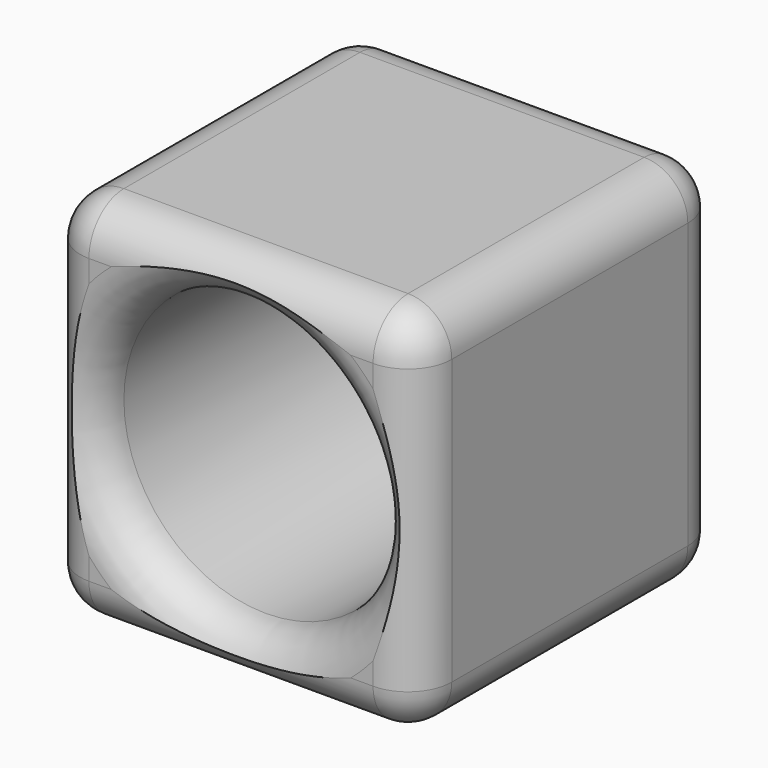
from build123d import *

# Parameters (mm, degrees)
F0_R         = 16.51
F1_DEPTH     = 6.35
F2_DEPTH     = 44.45
F3_T1_DEPTH  = 34.29
F3_T3_DEPTH  = 33.02
F3_T5_DEPTH  = 33.02
F3_S9_W      = 5.08
F3_S9_H      = 5.08
F3_T10_DEPTH = 5.08
F3_S15_W     = 5.08
F3_S15_H     = 5.08
F3_T16_DEPTH = 5.08
F3_S21_W     = 5.08
F3_S21_H     = 5.08
F3_T22_DEPTH = 5.08
F3_S27_W     = 5.08
F3_S27_H     = 5.08
F3_T28_DEPTH = 5.08
F3_S33_W     = 5.08
F3_S33_H     = 5.08
F3_T34_DEPTH = 5.08
F3_S39_W     = 5.08
F3_S39_H     = 5.08
F3_T40_DEPTH = 5.08
F3_S45_W     = 5.08
F3_S45_H     = 5.08
F3_T46_DEPTH = 5.08
F3_S51_W     = 5.08
F3_S51_H     = 5.08
F3_T52_DEPTH = 5.08
F4_R         = 3.175
F5_DEPTH     = 25.4


# Not quite as in the source:
# - a fillet or chamfer that OpenCascade refuses, or shapes differently, is made with other operations: its cross-section is extruded or revolved along the edge and cut away or added


with BuildPart() as f1:
    # F0 (on Front) → F1 (new body)
    with BuildSketch(Plane.XZ):
        Circle(F0_R)
    extrude(amount=F1_DEPTH)

    # F0 (on Front) → F2 (join)
    with BuildSketch(Plane.XZ):
        Polygon((21.59, 21.59), (0, 21.59), (-21.59, 21.59), (-21.59, 0), (-21.59, -21.59), (21.59, -21.59), align=None)
        Circle(F0_R, mode=Mode.SUBTRACT)
    extrude(amount=F2_DEPTH)

    # F3: fillet of radius 5.08 on 13 edges, made by hand

    # F3_s2 → F3_t1 (cut)
    with BuildSketch(Plane.XZ.offset(5.08)):
        with BuildLine():
            ThreePointArc((16.51, 21.59), (20.1021024484, 20.1021024484), (21.59, 16.51))
            Line((21.59, 16.51), (21.59, 21.59))
            Line((21.59, 21.59), (16.51, 21.59))
        make_face()
        with BuildLine():
            ThreePointArc((-16.51, 21.59), (-20.1021024484, 20.1021024484), (-21.59, 16.51))
            Line((-21.59, 16.51), (-21.59, 21.59))
            Line((-21.59, 21.59), (-16.51, 21.59))
        make_face()
        with BuildLine():
            ThreePointArc((-21.59, -16.51), (-20.1021024484, -20.1021024484), (-16.51, -21.59))
            Line((-16.51, -21.59), (-21.59, -21.59))
            Line((-21.59, -21.59), (-21.59, -16.51))
        make_face()
        with BuildLine():
            ThreePointArc((16.51, -21.59), (20.1021024484, -20.1021024484), (21.59, -16.51))
            Line((21.59, -16.51), (21.59, -21.59))
            Line((21.59, -21.59), (16.51, -21.59))
        make_face()
    extrude(amount=F3_T1_DEPTH, mode=Mode.SUBTRACT)

    # F3_s4 → F3_t3 (cut)
    with BuildSketch(Plane.YZ.offset(-16.51)):
        with BuildLine():
            ThreePointArc((0, -16.51), (-1.4878975516, -20.1021024484), (-5.08, -21.59))
            Line((-5.08, -21.59), (0, -21.59))
            Line((0, -21.59), (0, -16.51))
        make_face()
        with BuildLine():
            ThreePointArc((0, 16.51), (-1.4878975516, 20.1021024484), (-5.08, 21.59))
            Line((-5.08, 21.59), (0, 21.59))
            Line((0, 21.59), (0, 16.51))
        make_face()
        with BuildLine():
            ThreePointArc((-39.37, -21.59), (-42.9621024484, -20.1021024484), (-44.45, -16.51))
            Line((-44.45, -16.51), (-44.45, -21.59))
            Line((-44.45, -21.59), (-39.37, -21.59))
        make_face()
        with BuildLine():
            ThreePointArc((-39.37, 21.59), (-42.9621024484, 20.1021024484), (-44.45, 16.51))
            Line((-44.45, 16.51), (-44.45, 21.59))
            Line((-44.45, 21.59), (-39.37, 21.59))
        make_face()
    extrude(amount=F3_T3_DEPTH, mode=Mode.SUBTRACT)

    # F3_s6 → F3_t5 (cut)
    with BuildSketch(Plane.XY.offset(-16.51)):
        with BuildLine():
            ThreePointArc((16.51, 0), (20.1021024484, -1.4878975516), (21.59, -5.08))
            Line((21.59, -5.08), (21.59, 0))
            Line((21.59, 0), (16.51, 0))
        make_face()
        with BuildLine():
            ThreePointArc((-16.51, 0), (-20.1021024484, -1.4878975516), (-21.59, -5.08))
            Line((-21.59, -5.08), (-21.59, 0))
            Line((-21.59, 0), (-16.51, 0))
        make_face()
        with BuildLine():
            ThreePointArc((21.59, -39.37), (20.1021024484, -42.9621024484), (16.51, -44.45))
            Line((16.51, -44.45), (21.59, -44.45))
            Line((21.59, -44.45), (21.59, -39.37))
        make_face()
        with BuildLine():
            ThreePointArc((-21.59, -39.37), (-20.1021024484, -42.9621024484), (-16.51, -44.45))
            Line((-16.51, -44.45), (-21.59, -44.45))
            Line((-21.59, -44.45), (-21.59, -39.37))
        make_face()
    extrude(amount=F3_T5_DEPTH, mode=Mode.SUBTRACT)


with BuildPart() as f3_tool8:
    # F3_s9 → F3_t10 (new body)
    with BuildSketch(Plane.XZ.offset(5.08)):
        with Locations((19.05, 19.05)):
            Rectangle(F3_S9_W, F3_S9_H)
    extrude(amount=-F3_T10_DEPTH)

    # F3_s11 → F3_t12 (revolve, cut)
    with BuildSketch(Plane(origin=(16.51, -5.08, 16.51), x_dir=(-0.7071067812, 0, -0.7071067812), z_dir=(0.7071067812, 0, -0.7071067812))):
        with BuildLine():
            ThreePointArc((0, -5.08), (5.08, 0), (0, 5.08))
            Line((0, 5.08), (0, -5.08))
        make_face()
    revolve(axis=Axis((16.51, -5.08, 16.51), (0, 1, 0)), mode=Mode.SUBTRACT)


with BuildPart() as f1_1:
    add(f1.part)

    # F3_t7: cut F3_tool8
    add(f3_tool8.part, mode=Mode.SUBTRACT)


with BuildPart() as f3_tool14:
    # F3_s15 → F3_t16 (new body)
    with BuildSketch(Plane.XY.offset(16.51)):
        with Locations((19.05, -41.91)):
            Rectangle(F3_S15_W, F3_S15_H)
    extrude(amount=F3_T16_DEPTH)

    # F3_s17 → F3_t18 (revolve, cut)
    with BuildSketch(Plane(origin=(16.51, -39.37, 16.51), x_dir=(-0.7071067812, 0.7071067812, 0), z_dir=(0.7071067812, 0.7071067812, 0))):
        with BuildLine():
            ThreePointArc((0, -5.08), (5.08, 0), (0, 5.08))
            Line((0, 5.08), (0, -5.08))
        make_face()
    revolve(axis=Axis((16.51, -39.37, 16.51), (0, 0, 1)), mode=Mode.SUBTRACT)


with BuildPart() as f1_2:
    add(f1_1.part)

    # F3_t13: cut F3_tool14
    add(f3_tool14.part, mode=Mode.SUBTRACT)


with BuildPart() as f3_tool20:
    # F3_s21 → F3_t22 (new body)
    with BuildSketch(Plane.XZ.offset(5.08)):
        with Locations((-19.05, 19.05)):
            Rectangle(F3_S21_W, F3_S21_H)
    extrude(amount=-F3_T22_DEPTH)

    # F3_s23 → F3_t24 (revolve, cut)
    with BuildSketch(Plane(origin=(-16.51, -5.08, 16.51), x_dir=(0.7071067812, 0, -0.7071067812), z_dir=(0.7071067812, 0, 0.7071067812))):
        with BuildLine():
            ThreePointArc((0, -5.08), (5.08, 0), (0, 5.08))
            Line((0, 5.08), (0, -5.08))
        make_face()
    revolve(axis=Axis((-16.51, -5.08, 16.51), (0, 1, 0)), mode=Mode.SUBTRACT)


with BuildPart() as f1_3:
    add(f1_2.part)

    # F3_t19: cut F3_tool20
    add(f3_tool20.part, mode=Mode.SUBTRACT)


with BuildPart() as f3_tool26:
    # F3_s27 → F3_t28 (new body)
    with BuildSketch(Plane.XY.offset(16.51)):
        with Locations((-19.05, -41.91)):
            Rectangle(F3_S27_W, F3_S27_H)
    extrude(amount=F3_T28_DEPTH)

    # F3_s29 → F3_t30 (revolve, cut)
    with BuildSketch(Plane(origin=(-16.51, -39.37, 16.51), x_dir=(0.7071067812, 0.7071067812, 0), z_dir=(0.7071067812, -0.7071067812, 0))):
        with BuildLine():
            ThreePointArc((0, -5.08), (5.08, 0), (0, 5.08))
            Line((0, 5.08), (0, -5.08))
        make_face()
    revolve(axis=Axis((-16.51, -39.37, 16.51), (0, 0, 1)), mode=Mode.SUBTRACT)


with BuildPart() as f1_4:
    add(f1_3.part)

    # F3_t25: cut F3_tool26
    add(f3_tool26.part, mode=Mode.SUBTRACT)


with BuildPart() as f3_tool32:
    # F3_s33 → F3_t34 (new body)
    with BuildSketch(Plane.XZ.offset(5.08)):
        with Locations((-19.05, -19.05)):
            Rectangle(F3_S33_W, F3_S33_H)
    extrude(amount=-F3_T34_DEPTH)

    # F3_s35 → F3_t36 (revolve, cut)
    with BuildSketch(Plane(origin=(-16.51, -5.08, -16.51), x_dir=(0.7071067812, 0, 0.7071067812), z_dir=(-0.7071067812, 0, 0.7071067812))):
        with BuildLine():
            ThreePointArc((0, -5.08), (5.08, 0), (0, 5.08))
            Line((0, 5.08), (0, -5.08))
        make_face()
    revolve(axis=Axis((-16.51, -5.08, -16.51), (0, 1, 0)), mode=Mode.SUBTRACT)


with BuildPart() as f1_5:
    add(f1_4.part)

    # F3_t31: cut F3_tool32
    add(f3_tool32.part, mode=Mode.SUBTRACT)


with BuildPart() as f3_tool38:
    # F3_s39 → F3_t40 (new body)
    with BuildSketch(Plane.YZ.offset(-16.51)):
        with Locations((-41.91, -19.05)):
            Rectangle(F3_S39_W, F3_S39_H)
    extrude(amount=-F3_T40_DEPTH)

    # F3_s41 → F3_t42 (revolve, cut)
    with BuildSketch(Plane(origin=(-16.51, -39.37, -16.51), x_dir=(0, 0.7071067812, 0.7071067812), z_dir=(0, -0.7071067812, 0.7071067812))):
        with BuildLine():
            ThreePointArc((0, -5.08), (5.08, 0), (0, 5.08))
            Line((0, 5.08), (0, -5.08))
        make_face()
    revolve(axis=Axis((-16.51, -39.37, -16.51), (-1, 0, 0)), mode=Mode.SUBTRACT)


with BuildPart() as f1_6:
    add(f1_5.part)

    # F3_t37: cut F3_tool38
    add(f3_tool38.part, mode=Mode.SUBTRACT)


with BuildPart() as f3_tool44:
    # F3_s45 → F3_t46 (new body)
    with BuildSketch(Plane.XZ.offset(5.08)):
        with Locations((19.05, -19.05)):
            Rectangle(F3_S45_W, F3_S45_H)
    extrude(amount=-F3_T46_DEPTH)

    # F3_s47 → F3_t48 (revolve, cut)
    with BuildSketch(Plane(origin=(16.51, -5.08, -16.51), x_dir=(-0.7071067812, 0, 0.7071067812), z_dir=(-0.7071067812, 0, -0.7071067812))):
        with BuildLine():
            ThreePointArc((0, -5.08), (5.08, 0), (0, 5.08))
            Line((0, 5.08), (0, -5.08))
        make_face()
    revolve(axis=Axis((16.51, -5.08, -16.51), (0, 1, 0)), mode=Mode.SUBTRACT)


with BuildPart() as f1_7:
    add(f1_6.part)

    # F3_t43: cut F3_tool44
    add(f3_tool44.part, mode=Mode.SUBTRACT)


with BuildPart() as f3_tool50:
    # F3_s51 → F3_t52 (new body)
    with BuildSketch(Plane.XY.offset(-16.51)):
        with Locations((19.05, -41.91)):
            Rectangle(F3_S51_W, F3_S51_H)
    extrude(amount=-F3_T52_DEPTH)

    # F3_s53 → F3_t54 (revolve, cut)
    with BuildSketch(Plane(origin=(16.51, -39.37, -16.51), x_dir=(-0.7071067812, 0.7071067812, 0), z_dir=(-0.7071067812, -0.7071067812, 0))):
        with BuildLine():
            ThreePointArc((0, -5.08), (5.08, 0), (0, 5.08))
            Line((0, 5.08), (0, -5.08))
        make_face()
    revolve(axis=Axis((16.51, -39.37, -16.51), (0, 0, -1)), mode=Mode.SUBTRACT)


with BuildPart() as f1_8:
    add(f1_7.part)

    # F3_t49: cut F3_tool50
    add(f3_tool50.part, mode=Mode.SUBTRACT)

    # F3_s55 → F3_t56 (revolve, cut)
    with BuildSketch(Plane.XY):
        with BuildLine():
            ThreePointArc((21.59, -44.45), (17.9978975516, -42.9621024484), (16.51, -39.37))
            Line((16.51, -39.37), (16.51, -44.45))
            Line((16.51, -44.45), (21.59, -44.45))
        make_face()
    revolve(axis=Axis((0, -44.45, 0), (0, -1, 0)), mode=Mode.SUBTRACT)

    # F4 (on face) → F5 (cut)
    with BuildSketch(Plane(origin=(0, 0, 0), x_dir=(-1, 0, 0), z_dir=(0, 1, 0))):
        with Locations((-8.255, 0)):
            Circle(F4_R)
        with Locations((8.255, 0)):
            Circle(F4_R)
    extrude(amount=-F5_DEPTH, mode=Mode.SUBTRACT)


solid = f1_8.part
